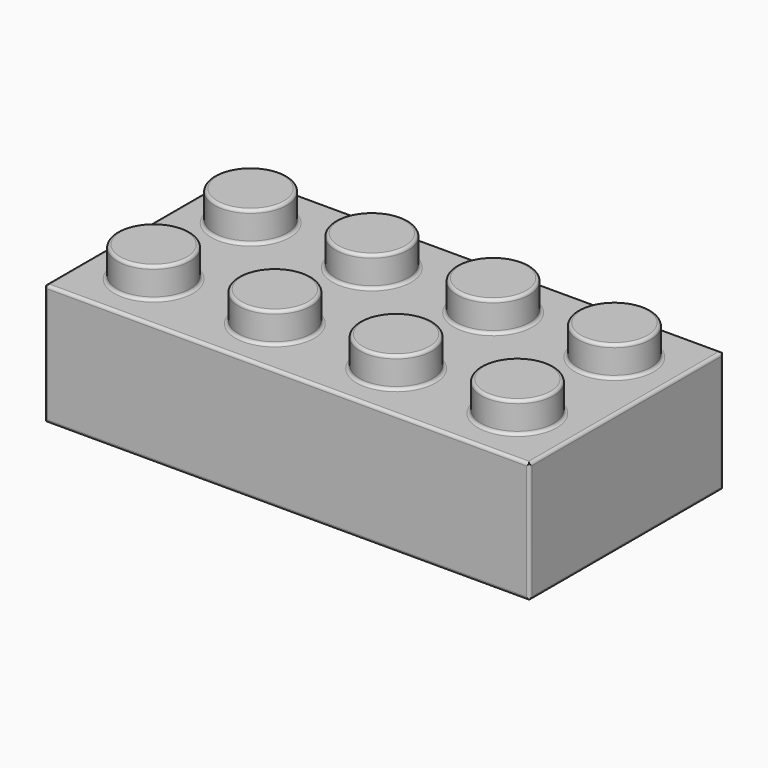
from build123d import *

# Parameters (mm, degrees)
F0_W          = 160
F0_H          = 80
F1_DEPTH      = 40
F2_W          = 144
F2_H          = 64
F3_DEPTH      = 30
F4_R          = 12
F5_DEPTH      = 10
F6_R          = 1
F7_R          = 1
F8_T1_DEPTH   = 44
F8_T3_DEPTH   = 165
F9_T1_DEPTH   = 44
F9_T3_DEPTH   = 84
F10_T1_DEPTH  = 84
F10_T3_DEPTH  = 44
F11_T1_DEPTH  = 163
F11_T3_DEPTH  = 144
F11_T5_DEPTH  = 64
F11_T11_DEPTH = 146.5
F11_T15_DEPTH = 66.5
F11_T22_DEPTH = 146.5
F11_T26_DEPTH = 66.5
F11_T33_DEPTH = 66.5
F11_T37_DEPTH = 146.5
F11_T44_DEPTH = 66.5
F11_T48_DEPTH = 146.5


# Not quite as in the source:
# - a fillet or chamfer that OpenCascade refuses, or shapes differently, is made with other operations: its cross-section is extruded or revolved along the edge and cut away or added


with BuildPart() as f1:
    # F0 (on Top) → F1 (new body)
    with BuildSketch(Plane.XY):
        with Locations((4.6006888151, 1.4286273053)):
            Rectangle(F0_W, F0_H)
    extrude(amount=F1_DEPTH)

    # F2 (on face) → F3 (cut)
    with BuildSketch(Plane(origin=(0, 0, 0), x_dir=(1, 0, 0), z_dir=(0, 0, -1))):
        with Locations((4.6006888151, -1.4286273053)):
            Rectangle(F2_W, F2_H)
    extrude(amount=-F3_DEPTH, mode=Mode.SUBTRACT)

    # F4 (on face) → F5 (join)
    with BuildSketch(Plane.XY.offset(40)):
        with Locations((-55.3993111849, 21.4286273053)):
            Circle(F4_R)
        with Locations((-15.3993111849, 21.4286273053)):
            Circle(F4_R)
        with Locations((24.6006888151, 21.4286273053)):
            Circle(F4_R)
        with Locations((64.6006888151, 21.4286273053)):
            Circle(F4_R)
        with Locations((-55.3993111849, -18.5713726947)):
            Circle(F4_R)
        with Locations((-15.3993111849, -18.5713726947)):
            Circle(F4_R)
        with Locations((24.6006888151, -18.5713726947)):
            Circle(F4_R)
        with Locations((64.6006888151, -18.5713726947)):
            Circle(F4_R)
    extrude(amount=F5_DEPTH)

    # F6
    f6_edges = [f1.edges().sort_by_distance(p)[0] for p in [
        (-67.399311, 21.428627, 50),
        (-27.399311, 21.428627, 50),
        (-67.399311, -18.571373, 50),
        (-27.399311, -18.571373, 50),
        (12.600689, 21.428627, 50),
        (52.600689, 21.428627, 50),
        (52.600689, -18.571373, 50),
        (12.600689, -18.571373, 50),
    ]]
    fillet(f6_edges, radius=F6_R)

    # F7
    f7_edges = [f1.edges().sort_by_distance(p)[0] for p in [
        (4.600689, 41.428627, 40),
        (84.600689, 1.428627, 40),
        (-75.399311, 1.428627, 40),
        (4.600689, -38.571373, 40),
        (-67.399311, -18.571373, 40),
        (-27.399311, -18.571373, 40),
        (12.600689, -18.571373, 40),
        (52.600689, -18.571373, 40),
        (-67.399311, 21.428627, 40),
        (-27.399311, 21.428627, 40),
        (12.600689, 21.428627, 40),
        (52.600689, 21.428627, 40),
    ]]
    fillet(f7_edges, radius=F7_R)

    # F8: fillet of radius 1 on 4 edges, made by hand

    # F8_s2 → F8_t1 (cut)
    with BuildSketch(Plane.XY.offset(-2.5)):
        with BuildLine():
            ThreePointArc((-75.3993111849, -37.5713726947), (-75.1064179661, -38.2784794759), (-74.3993111849, -38.5713726947))
            Line((-74.3993111849, -38.5713726947), (-75.3993111849, -38.5713726947))
            Line((-75.3993111849, -38.5713726947), (-75.3993111849, -37.5713726947))
        make_face()
        with BuildLine():
            ThreePointArc((84.6006888151, -37.5713726947), (84.3077955963, -38.2784794759), (83.6006888151, -38.5713726947))
            Line((83.6006888151, -38.5713726947), (84.6006888151, -38.5713726947))
            Line((84.6006888151, -38.5713726947), (84.6006888151, -37.5713726947))
        make_face()
    extrude(amount=F8_T1_DEPTH, mode=Mode.SUBTRACT)

    # F8_s4 → F8_t3 (cut)
    with BuildSketch(Plane.YZ.offset(-77.8993111849)):
        with BuildLine():
            ThreePointArc((-38.5713726947, 1), (-38.2784794759, 0.2928932188), (-37.5713726947, 0))
            Line((-37.5713726947, 0), (-38.5713726947, 0))
            Line((-38.5713726947, 0), (-38.5713726947, 1))
        make_face()
    extrude(amount=F8_T3_DEPTH, mode=Mode.SUBTRACT)

    # F9: fillet of radius 1 on 4 edges, made by hand

    # F9_s2 → F9_t1 (cut)
    with BuildSketch(Plane.XY.offset(-2.5)):
        with BuildLine():
            ThreePointArc((-74.3993111849, 41.4286273053), (-75.1064179661, 41.1357340865), (-75.3993111849, 40.4286273053))
            Line((-75.3993111849, 40.4286273053), (-75.3993111849, 41.4286273053))
            Line((-75.3993111849, 41.4286273053), (-74.3993111849, 41.4286273053))
        make_face()
    extrude(amount=F9_T1_DEPTH, mode=Mode.SUBTRACT)

    # F9_s4 → F9_t3 (cut)
    with BuildSketch(Plane.XZ.offset(-43.9286273053)):
        with BuildLine():
            ThreePointArc((-75.3993111849, 1), (-75.1064179661, 0.2928932188), (-74.3993111849, 0))
            Line((-74.3993111849, 0), (-75.3993111849, 0))
            Line((-75.3993111849, 0), (-75.3993111849, 1))
        make_face()
    extrude(amount=F9_T3_DEPTH, mode=Mode.SUBTRACT)

    # F10: fillet of radius 1 on 4 edges, made by hand

    # F10_s2 → F10_t1 (cut)
    with BuildSketch(Plane.XZ.offset(-43.9286273053)):
        with BuildLine():
            ThreePointArc((84.6006888151, 1), (84.3077955963, 0.2928932188), (83.6006888151, 0))
            Line((83.6006888151, 0), (84.6006888151, 0))
            Line((84.6006888151, 0), (84.6006888151, 1))
        make_face()
    extrude(amount=F10_T1_DEPTH, mode=Mode.SUBTRACT)

    # F10_s4 → F10_t3 (cut)
    with BuildSketch(Plane.XY.offset(-2.5)):
        with BuildLine():
            ThreePointArc((83.6006888151, 41.4286273053), (84.3077955963, 41.1357340865), (84.6006888151, 40.4286273053))
            Line((84.6006888151, 40.4286273053), (84.6006888151, 41.4286273053))
            Line((84.6006888151, 41.4286273053), (83.6006888151, 41.4286273053))
        make_face()
    extrude(amount=F10_T3_DEPTH, mode=Mode.SUBTRACT)

    # F11: fillet of radius 1 on 8 edges, made by hand

    # F11_s2 → F11_t1 (cut)
    with BuildSketch(Plane.YZ.offset(-76.8993111849)):
        with BuildLine():
            ThreePointArc((41.4286273053, 1), (41.1357340865, 0.2928932188), (40.4286273053, 0))
            Line((40.4286273053, 0), (41.4286273053, 0))
            Line((41.4286273053, 0), (41.4286273053, 1))
        make_face()
    extrude(amount=F11_T1_DEPTH, mode=Mode.SUBTRACT)

    # F11_s4 → F11_t3 (cut)
    with BuildSketch(Plane.YZ.offset(-67.3993111849)):
        with BuildLine():
            ThreePointArc((34.4286273053, 0), (33.7215205241, 0.2928932188), (33.4286273053, 1))
            Line((33.4286273053, 1), (33.4286273053, 0))
            Line((33.4286273053, 0), (34.4286273053, 0))
        make_face()
        with BuildLine():
            ThreePointArc((-31.5713726947, 0), (-30.8642659135, 0.2928932188), (-30.5713726947, 1))
            Line((-30.5713726947, 1), (-30.5713726947, 0))
            Line((-30.5713726947, 0), (-31.5713726947, 0))
        make_face()
    extrude(amount=F11_T3_DEPTH, mode=Mode.SUBTRACT)

    # F11_s6 → F11_t5 (cut)
    with BuildSketch(Plane.XZ.offset(-33.4286273053)):
        with BuildLine():
            ThreePointArc((-68.3993111849, 0), (-67.6922044037, 0.2928932188), (-67.3993111849, 1))
            Line((-67.3993111849, 1), (-67.3993111849, 0))
            Line((-67.3993111849, 0), (-68.3993111849, 0))
        make_face()
        with BuildLine():
            ThreePointArc((77.6006888151, 0), (76.8935820339, 0.2928932188), (76.6006888151, 1))
            Line((76.6006888151, 1), (76.6006888151, 0))
            Line((76.6006888151, 0), (77.6006888151, 0))
        make_face()
    extrude(amount=F11_T5_DEPTH, mode=Mode.SUBTRACT)


with BuildPart() as f11_tool9:
    # F11_s10 → F11_t11 (new body)
    with BuildSketch(Plane.YZ.offset(-69.8993111849)):
        with BuildLine():
            ThreePointArc((34.4286273053, 0), (33.7215205241, 0.2928932188), (33.4286273053, 1))
            Line((33.4286273053, 1), (33.4286273053, 0))
            Line((33.4286273053, 0), (34.4286273053, 0))
        make_face()
    extrude(amount=F11_T11_DEPTH)

    split(bisect_by=Plane.YZ.offset(-67.3993111849), keep=Keep.BOTTOM)


with BuildPart() as f11_tool13:
    # F11_s14 → F11_t15 (new body)
    with BuildSketch(Plane.XZ.offset(30.5713726947)):
        with BuildLine():
            ThreePointArc((-68.3993111849, 0), (-67.6922044037, 0.2928932188), (-67.3993111849, 1))
            Line((-67.3993111849, 1), (-67.3993111849, 0))
            Line((-67.3993111849, 0), (-68.3993111849, 0))
        make_face()
    extrude(amount=-F11_T15_DEPTH)

    split(bisect_by=Plane.XZ.offset(-33.4286273053), keep=Keep.BOTTOM)


with BuildPart() as f11_tool9_1:
    add(f11_tool9.part)

    # F11_t17: intersect F11_tool13
    add(f11_tool13.part, mode=Mode.INTERSECT)


with BuildPart() as f1_1:
    add(f1.part)

    # F11_t7: cut F11_tool9
    add(f11_tool9_1.part, mode=Mode.SUBTRACT)


with BuildPart() as f11_tool20:
    # F11_s21 → F11_t22 (new body)
    with BuildSketch(Plane.YZ.offset(-67.3993111849)):
        with BuildLine():
            ThreePointArc((34.4286273053, 0), (33.7215205241, 0.2928932188), (33.4286273053, 1))
            Line((33.4286273053, 1), (33.4286273053, 0))
            Line((33.4286273053, 0), (34.4286273053, 0))
        make_face()
    extrude(amount=F11_T22_DEPTH)

    split(bisect_by=Plane.YZ.offset(76.6006888151), keep=Keep.TOP)


with BuildPart() as f11_tool24:
    # F11_s25 → F11_t26 (new body)
    with BuildSketch(Plane.XZ.offset(-35.9286273053)):
        with BuildLine():
            ThreePointArc((77.6006888151, 0), (76.8935820339, 0.2928932188), (76.6006888151, 1))
            Line((76.6006888151, 1), (76.6006888151, 0))
            Line((76.6006888151, 0), (77.6006888151, 0))
        make_face()
    extrude(amount=F11_T26_DEPTH)

    split(bisect_by=Plane.XZ.offset(-33.4286273053), keep=Keep.BOTTOM)


with BuildPart() as f11_tool20_1:
    add(f11_tool20.part)

    # F11_t28: intersect F11_tool24
    add(f11_tool24.part, mode=Mode.INTERSECT)


with BuildPart() as f1_2:
    add(f1_1.part)

    # F11_t18: cut F11_tool20
    add(f11_tool20_1.part, mode=Mode.SUBTRACT)


with BuildPart() as f11_tool31:
    # F11_s32 → F11_t33 (new body)
    with BuildSketch(Plane.XZ.offset(33.0713726947)):
        with BuildLine():
            ThreePointArc((-68.3993111849, 0), (-67.6922044037, 0.2928932188), (-67.3993111849, 1))
            Line((-67.3993111849, 1), (-67.3993111849, 0))
            Line((-67.3993111849, 0), (-68.3993111849, 0))
        make_face()
    extrude(amount=-F11_T33_DEPTH)

    split(bisect_by=Plane.XZ.offset(30.5713726947), keep=Keep.TOP)


with BuildPart() as f11_tool35:
    # F11_s36 → F11_t37 (new body)
    with BuildSketch(Plane.YZ.offset(76.6006888151)):
        with BuildLine():
            ThreePointArc((-31.5713726947, 0), (-30.8642659135, 0.2928932188), (-30.5713726947, 1))
            Line((-30.5713726947, 1), (-30.5713726947, 0))
            Line((-30.5713726947, 0), (-31.5713726947, 0))
        make_face()
    extrude(amount=-F11_T37_DEPTH)

    split(bisect_by=Plane.YZ.offset(-67.3993111849), keep=Keep.BOTTOM)


with BuildPart() as f11_tool31_1:
    add(f11_tool31.part)

    # F11_t39: intersect F11_tool35
    add(f11_tool35.part, mode=Mode.INTERSECT)


with BuildPart() as f1_3:
    add(f1_2.part)

    # F11_t29: cut F11_tool31
    add(f11_tool31_1.part, mode=Mode.SUBTRACT)


with BuildPart() as f11_tool42:
    # F11_s43 → F11_t44 (new body)
    with BuildSketch(Plane.XZ.offset(-33.4286273053)):
        with BuildLine():
            ThreePointArc((77.6006888151, 0), (76.8935820339, 0.2928932188), (76.6006888151, 1))
            Line((76.6006888151, 1), (76.6006888151, 0))
            Line((76.6006888151, 0), (77.6006888151, 0))
        make_face()
    extrude(amount=F11_T44_DEPTH)

    split(bisect_by=Plane.XZ.offset(30.5713726947), keep=Keep.TOP)


with BuildPart() as f11_tool46:
    # F11_s47 → F11_t48 (new body)
    with BuildSketch(Plane.YZ.offset(79.1006888151)):
        with BuildLine():
            ThreePointArc((-31.5713726947, 0), (-30.8642659135, 0.2928932188), (-30.5713726947, 1))
            Line((-30.5713726947, 1), (-30.5713726947, 0))
            Line((-30.5713726947, 0), (-31.5713726947, 0))
        make_face()
    extrude(amount=-F11_T48_DEPTH)

    split(bisect_by=Plane.YZ.offset(76.6006888151), keep=Keep.TOP)


with BuildPart() as f11_tool42_1:
    add(f11_tool42.part)

    # F11_t50: intersect F11_tool46
    add(f11_tool46.part, mode=Mode.INTERSECT)


with BuildPart() as f1_4:
    add(f1_3.part)

    # F11_t40: cut F11_tool42
    add(f11_tool42_1.part, mode=Mode.SUBTRACT)


solid = f1_4.part
